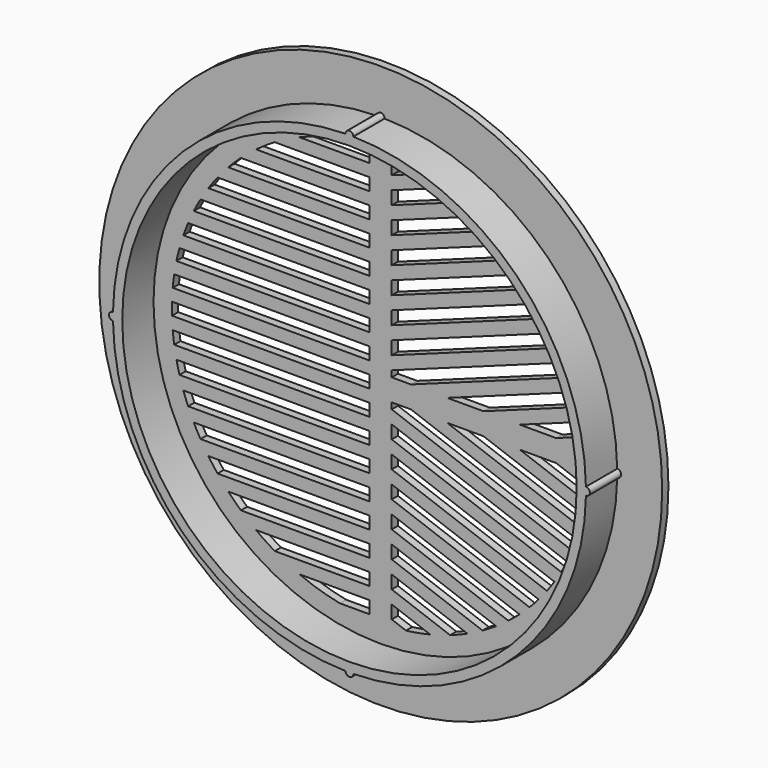
from build123d import *

# Parameters (mm, degrees)
F3_DEPTH      = 25
F2_R          = 58.1248774064
F4_DEPTH      = 2
F2_R_2        = 72
F5_DEPTH      = 10
F5_DEPTH_BACK = 2
F7_DEPTH      = 2


# Not quite as in the source:
# - ends of sketch curves that miss each other by under 0.0002 mm in the source are joined


with BuildPart() as f3:
    # F2 (on offset) → F3 (new body)
    with BuildSketch(Plane.XZ.offset(-10)):
        with BuildLine():
            Line((-2.8117546, -52.3882112), (-10.4651656881, -52.3882112))
            ThreePointArc((-10.4651656881, -52.3882112), (-2.0290554984, -53.3847103523), (6.4583568386, -53.0314434327))
            Line((6.4583568386, -53.0314434327), (2.8133294, -51.7046972))
            Line((2.8133294, -51.7046972), (2.8133294, -48.3271576))
            Line((2.8133294, -48.3271576), (12.6439208004, -51.9054489665))
            ThreePointArc((12.6439208004, -51.9054489665), (15.218427268, -51.2098021584), (17.7550108574, -50.3865453774))
            Line((17.7550108574, -50.3865453774), (2.8133294, -44.9481956))
            Line((2.8133294, -44.9481956), (2.8133294, -41.5692336))
            Line((2.8133294, -41.5692336), (22.1596901051, -48.610621268))
            ThreePointArc((22.1596901051, -48.610621268), (24.1217019206, -47.6674717398), (26.0436606582, -46.6451723669))
            Line((26.0436606582, -46.6451723669), (2.8133294, -38.1905256))
            Line((2.8133294, -38.1905256), (2.8133294, -34.8115636))
            Line((2.8133294, -34.8115636), (29.5155011347, -44.529535798))
            ThreePointArc((29.5155011347, -44.529535798), (31.0993092601, -43.4382012652), (32.6428059495, -42.2905614217))
            Line((32.6428059495, -42.2905614217), (2.8133294, -31.4323476))
            Line((2.8133294, -31.4323476), (2.8133294, -28.0533856))
            Line((2.8133294, -28.0533856), (35.4767217693, -39.9430416734))
            ThreePointArc((35.4767217693, -39.9430416734), (36.7835304475, -38.7429510161), (38.0497674642, -37.500127487))
            Line((38.0497674642, -37.500127487), (2.8133294, -24.6744236))
            Line((2.8133294, -24.6744236), (2.8133294, -21.2969856))
            Line((2.8133294, -21.2969856), (40.3860770749, -34.9715476368))
            ThreePointArc((40.3860770749, -34.9715476368), (41.4655782018, -33.6845690192), (42.5040845927, -32.3642883214))
            Line((42.5040845927, -32.3642883214), (2.8133294, -17.9180236))
            Line((2.8133294, -17.9180236), (2.8133294, -14.5390616))
            Line((2.8133294, -14.5390616), (44.4188112616, -29.6818727798))
            ThreePointArc((44.4188112616, -29.6818727798), (45.3001399367, -28.3185749524), (46.1396401032, -26.9291287784))
            Line((46.1396401032, -26.9291287784), (2.8133294, -11.1603536))
            Line((2.8133294, -11.1603536), (2.8133294, -7.7808836))
            Line((2.8133294, -7.7808836), (47.6735638969, -24.109659288))
            ThreePointArc((47.6735638969, -24.109659288), (48.3716674827, -22.6765550857), (49.0267027126, -21.2232605117))
            Line((49.0267027126, -21.2232605117), (2.8133294, -4.4021756))
            Line((2.8133294, -4.4021756), (2.8133294, -2.8131516))
            Line((2.8133294, -2.8131516), (7.7274674, -2.8131516))
            Line((7.7274674, -2.8131516), (50.2014340828, -18.271846695))
            ThreePointArc((50.2014340828, -18.271846695), (50.722459913, -16.7712976835), (51.1986446, -15.2559220219))
            Line((51.1986446, -15.2559220219), (17.0096434, -2.8131516))
            Line((17.0096434, -2.8131516), (26.2938514, -2.8131516))
            Line((26.2938514, -2.8131516), (52.0175000452, -12.1747301681))
            ThreePointArc((52.0175000452, -12.1747301681), (52.3597146995, -10.6068205513), (52.654680648, -9.0293394816))
            Line((52.654680648, -9.0293394816), (35.5760274, -2.8131516))
            Line((35.5760274, -2.8131516), (44.8599814, -2.8131516))
            Line((44.8599814, -2.8131516), (53.1059491143, -5.8139946928))
            ThreePointArc((53.1059491143, -5.8139946928), (53.3438708851, -2.9113235155), (53.4232567859, 0))
            ThreePointArc((53.4232567859, 0), (53.3438698733, 2.9113420537), (53.1059450733, 5.814031604))
            Line((53.1059450733, 5.814031604), (44.8599814, 2.8119324))
            Line((44.8599814, 2.8119324), (35.5760274, 2.8119324))
            Line((35.5760274, 2.8119324), (52.6549590226, 9.0277159873))
            ThreePointArc((52.6549590226, 9.0277159873), (52.3598738539, 10.6060348678), (52.0174900396, 12.1747729176))
            Line((52.0174900396, 12.1747729176), (26.2938514, 2.8119324))
            Line((26.2938514, 2.8119324), (17.0096434, 2.8119324))
            Line((17.0096434, 2.8119324), (51.1986319495, 15.2559644767))
            ThreePointArc((51.1986319495, 15.2559644767), (50.7224085028, 16.7714531659), (50.2013372139, 18.2721128376))
            Line((50.2013372139, 18.2721128376), (7.7274674, 2.8119324))
            Line((7.7274674, 2.8119324), (2.8133294, 2.8119324))
            Line((2.8133294, 2.8119324), (2.8133294, 4.4022264))
            Line((2.8133294, 4.4022264), (49.0268732907, 21.222866464))
            ThreePointArc((49.0268732907, 21.222866464), (48.3720536469, 22.6757313354), (47.6741912545, 24.1084187338))
            Line((47.6741912545, 24.1084187338), (2.8133294, 7.7811884))
            Line((2.8133294, 7.7811884), (2.8133294, 11.1598964))
            Line((2.8133294, 11.1598964), (46.1394942326, 26.9293787076))
            ThreePointArc((46.1394942326, 26.9293787076), (45.3001153405, 28.318614298), (44.4189204817, 29.6817093318))
            Line((44.4189204817, 29.6817093318), (2.8133294, 14.5388584))
            Line((2.8133294, 14.5388584), (2.8133294, 17.9178204))
            Line((2.8133294, 17.9178204), (42.5040547328, 32.3643275364))
            ThreePointArc((42.5040547328, 32.3643275364), (41.4655480706, 33.6846061106), (40.3860467755, 34.9715826274))
            Line((40.3860467755, 34.9715826274), (2.8133294, 21.2952584))
            Line((2.8133294, 21.2952584), (2.8133294, 24.6744744))
            Line((2.8133294, 24.6744744), (38.0499142876, 37.4999785109))
            ThreePointArc((38.0499142876, 37.4999785109), (36.783684661, 38.7428046013), (35.4768833619, 39.942898149))
            Line((35.4768833619, 39.942898149), (2.8133294, 28.0534364))
            Line((2.8133294, 28.0534364), (2.8133294, 31.4323984))
            Line((2.8133294, 31.4323984), (32.6429839509, 42.2904240271))
            ThreePointArc((32.6429839509, 42.2904240271), (31.0993770857, 43.4381527059), (29.5154527684, 44.5295678566))
            Line((29.5154527684, 44.5295678566), (2.8133294, 34.8113604))
            Line((2.8133294, 34.8113604), (2.8133294, 38.1903224))
            Line((2.8133294, 38.1903224), (26.04388098, 46.6450493527))
            ThreePointArc((26.04388098, 46.6450493527), (24.1219360197, 47.6673532753), (22.1599379618, 48.610508279))
            Line((22.1599379618, 48.610508279), (2.8133294, 41.5690304))
            Line((2.8133294, 41.5690304), (2.8133294, 44.9479924))
            Line((2.8133294, 44.9479924), (17.7553997833, 50.3864083276))
            ThreePointArc((17.7553997833, 50.3864083276), (15.2185413933, 51.2097682427), (12.643751501, 51.9054902067))
            Line((12.643751501, 51.9054902067), (2.8133294, 48.3259384))
            Line((2.8133294, 48.3259384), (2.8133294, 51.7046464))
            Line((2.8133294, 51.7046464), (6.4589618961, 53.0313697432))
            ThreePointArc((6.4589618961, 53.0313697432), (-2.0327661079, 53.3845691897), (-10.4730459901, 52.3866364))
            Line((-10.4730459901, 52.3866364), (-2.8117546, 52.3866364))
            Line((-2.8117546, 52.3866364), (-2.8117546, 49.2116364))
            Line((-2.8117546, 49.2116364), (-20.7908443419, 49.2116364))
            ThreePointArc((-20.7908443419, 49.2116364), (-24.0004032321, 47.728660261), (-27.104842272, 46.0366364))
            Line((-27.104842272, 46.0366364), (-2.8117546, 46.0366364))
            Line((-2.8117546, 46.0366364), (-2.8117546, 42.8616364))
            Line((-2.8117546, 42.8616364), (-31.8892535305, 42.8616364))
            ThreePointArc((-31.8892535305, 42.8616364), (-33.8635191157, 41.3195648418), (-35.7633227884, 39.6866364))
            Line((-35.7633227884, 39.6866364), (-2.8117546, 39.6866364))
            Line((-2.8117546, 39.6866364), (-2.8117546, 36.5116364))
            Line((-2.8117546, 36.5116364), (-38.9992919552, 36.5116364))
            ThreePointArc((-38.9992919552, 36.5116364), (-40.4037524944, 34.9511251605), (-41.7458146303, 33.3366364))
            Line((-41.7458146303, 33.3366364), (-2.8117546, 33.3366364))
            Line((-2.8117546, 33.3366364), (-2.8117546, 30.1616364))
            Line((-2.8117546, 30.1616364), (-44.0944447214, 30.1616364))
            ThreePointArc((-44.0944447214, 30.1616364), (-45.1281672323, 28.5918325377), (-46.1060280379, 26.9866364))
            Line((-46.1060280379, 26.9866364), (-2.8117546, 26.9866364))
            Line((-2.8117546, 26.9866364), (-2.8117546, 23.8116364))
            Line((-2.8117546, 23.8116364), (-47.8231150969, 23.8116364))
            ThreePointArc((-47.8231150969, 23.8116364), (-48.5757557209, 22.2360140709), (-49.2765015368, 20.6366364))
            Line((-49.2765015368, 20.6366364), (-2.8117546, 20.6366364))
            Line((-2.8117546, 20.6366364), (-2.8117546, 17.4616364))
            Line((-2.8117546, 17.4616364), (-50.4889653276, 17.4616364))
            ThreePointArc((-50.4889653276, 17.4616364), (-51.0079586216, 15.8818299598), (-51.4775328273, 14.2866364))
            Line((-51.4775328273, 14.2866364), (-2.8117546, 14.2866364))
            Line((-2.8117546, 14.2866364), (-2.8117546, 11.1116364))
            Line((-2.8117546, 11.1116364), (-52.2549127081, 11.1116364))
            ThreePointArc((-52.2549127081, 11.1116364), (-52.5666470955, 9.5284825), (-52.8304284316, 7.9366364))
            Line((-52.8304284316, 7.9366364), (-2.8117546, 7.9366364))
            Line((-2.8117546, 7.9366364), (-2.8117546, 4.7616364))
            Line((-2.8117546, 4.7616364), (-53.2106303704, 4.7616364))
            ThreePointArc((-53.2106303704, 4.7616364), (-53.3287941262, 3.1755444663), (-53.399690502, 1.5866379243))
            Line((-53.399690502, 1.5866379243), (-2.8117546, 1.5866364))
            Line((-2.8117546, 1.5866364), (-2.8117546, -1.5883636))
            Line((-2.8117546, -1.5883636), (-53.3996392, -1.5883636))
            ThreePointArc((-53.3996392, -1.5883636), (-53.3286912488, -3.1772716764), (-53.2104757809, -4.7633636))
            Line((-53.2104757809, -4.7633636), (-2.8117546, -4.7633636))
            Line((-2.8117546, -4.7633636), (-2.8117546, -7.9383636))
            Line((-2.8117546, -7.9383636), (-52.8301689281, -7.9383636))
            ThreePointArc((-52.8301689281, -7.9383636), (-52.5663338333, -9.53021054), (-52.2545454014, -11.1133636))
            Line((-52.2545454014, -11.1133636), (-2.8117546, -11.1133636))
            Line((-2.8117546, -11.1133636), (-2.8117546, -14.2883636))
            Line((-2.8117546, -14.2883636), (-51.4770534437, -14.2883636))
            ThreePointArc((-51.4770534437, -14.2883636), (-51.0074204976, -15.8835581593), (-50.4883679414, -17.4633636))
            Line((-50.4883679414, -17.4633636), (-2.8117546, -17.4633636))
            Line((-2.8117546, -17.4633636), (-2.8117546, -20.6383636))
            Line((-2.8117546, -20.6383636), (-49.2757781626, -20.6383636))
            ThreePointArc((-49.2757781626, -20.6383636), (-48.5749644416, -22.2377425813), (-47.8222550668, -23.8133636))
            Line((-47.8222550668, -23.8133636), (-2.8117546, -23.8133636))
            Line((-2.8117546, -23.8133636), (-2.8117546, -26.9883636))
            Line((-2.8117546, -26.9883636), (-46.1050170351, -26.9883636))
            ThreePointArc((-46.1050170351, -26.9883636), (-45.127071662, -28.5935616675), (-44.0932632264, -30.1633636))
            Line((-44.0932632264, -30.1633636), (-2.8117546, -30.1633636))
            Line((-2.8117546, -30.1633636), (-2.8117546, -33.3383636))
            Line((-2.8117546, -33.3383636), (-41.7444352949, -33.3383636))
            ThreePointArc((-41.7444352949, -33.3383636), (-40.4022554344, -34.9528556978), (-38.9976748567, -36.5133636))
            Line((-38.9976748567, -36.5133636), (-2.8117546, -36.5133636))
            Line((-2.8117546, -36.5133636), (-2.8117546, -39.6881096))
            Line((-2.8117546, -39.6881096), (-35.7616879075, -39.6881096))
            ThreePointArc((-35.7616879075, -39.6881096), (-33.8617135671, -41.3210445162), (-31.8872733396, -42.8631096))
            Line((-31.8872733396, -42.8631096), (-2.8117546, -42.8631096))
            Line((-2.8117546, -42.8631096), (-2.8117546, -46.0381096))
            Line((-2.8117546, -46.0381096), (-27.1023399373, -46.0381096))
            ThreePointArc((-27.1023399373, -46.0381096), (-23.9972982866, -47.7302214594), (-20.7871164186, -49.2132112))
            Line((-20.7871164186, -49.2132112), (-2.8117546, -49.2132112))
            Line((-2.8117546, -49.2132112), (-2.8117546, -52.3882112))
        make_face()
    extrude(amount=F3_DEPTH)


with BuildPart() as f4:
    # F2 (on offset) → F4 (new body)
    with BuildSketch(Plane.XZ.offset(-10)):
        Circle(F2_R)
        with BuildLine():
            ThreePointArc((6.4583568386, -53.0314434327), (-2.0290554984, -53.3847103523), (-10.4651656881, -52.3882112))
            ThreePointArc((-10.4651656881, -52.3882112), (-15.7065731612, -51.0621966346), (-20.7871164186, -49.2132112))
            ThreePointArc((-20.7871164186, -49.2132112), (-23.9972982866, -47.7302214594), (-27.1023399373, -46.0381096))
            ThreePointArc((-27.1023399373, -46.0381096), (-29.5374977764, -44.514947947), (-31.8872733396, -42.8631096))
            ThreePointArc((-31.8872733396, -42.8631096), (-33.8617135671, -41.3210445162), (-35.7616879075, -39.6881096))
            ThreePointArc((-35.7616879075, -39.6881096), (-37.4133710493, -38.1350761419), (-38.9976748567, -36.5133636))
            ThreePointArc((-38.9976748567, -36.5133636), (-40.4022554344, -34.9528556978), (-41.7444352949, -33.3383636))
            ThreePointArc((-41.7444352949, -33.3383636), (-42.9481987761, -31.7725760288), (-44.0932632264, -30.1633636))
            ThreePointArc((-44.0932632264, -30.1633636), (-45.127071662, -28.5935616675), (-46.1050170351, -26.9883636))
            ThreePointArc((-46.1050170351, -26.9883636), (-46.9904593229, -25.4153712985), (-47.8222550668, -23.8133636))
            ThreePointArc((-47.8222550668, -23.8133636), (-48.5749644416, -22.2377425813), (-49.2757781626, -20.6383636))
            ThreePointArc((-49.2757781626, -20.6383636), (-49.9073278008, -19.0605088442), (-50.4883679414, -17.4633636))
            ThreePointArc((-50.4883679414, -17.4633636), (-51.0074204976, -15.8835581593), (-51.4770534437, -14.2883636))
            ThreePointArc((-51.4770534437, -14.2883636), (-51.8900887067, -12.7068115443), (-52.2545454014, -11.1133636))
            ThreePointArc((-52.2545454014, -11.1133636), (-52.5663338333, -9.53021054), (-52.8301689281, -7.9383636))
            ThreePointArc((-52.8301689281, -7.9383636), (-53.0440829766, -6.3537096874), (-53.2104757809, -4.7633636))
            ThreePointArc((-53.2104757809, -4.7633636), (-53.3286912488, -3.1772716764), (-53.3996392, -1.5883636))
            ThreePointArc((-53.3996392, -1.5883636), (-53.423256779, -0.000863219), (-53.399690502, 1.5866379243))
            ThreePointArc((-53.399690502, 1.5866379243), (-53.3287941262, 3.1755444663), (-53.2106303704, 4.7616364))
            ThreePointArc((-53.2106303704, 4.7616364), (-53.0442899303, 6.3519816911), (-52.8304284316, 7.9366364))
            ThreePointArc((-52.8304284316, 7.9366364), (-52.5666470955, 9.5284825), (-52.2549127081, 11.1116364))
            ThreePointArc((-52.2549127081, 11.1116364), (-51.8905118537, 12.7050834384), (-51.4775328273, 14.2866364))
            ThreePointArc((-51.4775328273, 14.2866364), (-51.0079586216, 15.8818299598), (-50.4889653276, 17.4616364))
            ThreePointArc((-50.4889653276, 17.4616364), (-49.9079878468, 19.0587805144), (-49.2765015368, 20.6366364))
            ThreePointArc((-49.2765015368, 20.6366364), (-48.5757557209, 22.2360140709), (-47.8231150969, 23.8116364))
            ThreePointArc((-47.8231150969, 23.8116364), (-46.9913943053, 25.4136425342), (-46.1060280379, 26.9866364))
            ThreePointArc((-46.1060280379, 26.9866364), (-45.1281672323, 28.5918325377), (-44.0944447214, 30.1616364))
            ThreePointArc((-44.0944447214, 30.1616364), (-42.9494783163, 31.7708463528), (-41.7458146303, 33.3366364))
            ThreePointArc((-41.7458146303, 33.3366364), (-40.4037524944, 34.9511251605), (-38.9992919552, 36.5116364))
            ThreePointArc((-38.9992919552, 36.5116364), (-37.4150009632, 38.1334770056), (-35.7633227884, 39.6866364))
            ThreePointArc((-35.7633227884, 39.6866364), (-33.8635191157, 41.3195648418), (-31.8892535305, 42.8616364))
            ThreePointArc((-31.8892535305, 42.8616364), (-29.5397358001, 44.5134628453), (-27.104842272, 46.0366364))
            ThreePointArc((-27.104842272, 46.0366364), (-24.0004032321, 47.728660261), (-20.7908443419, 49.2116364))
            ThreePointArc((-20.7908443419, 49.2116364), (-15.7123475624, 51.0604200893), (-10.4730459901, 52.3866364))
            ThreePointArc((-10.4730459901, 52.3866364), (-2.0327661079, 53.3845691897), (6.4589618961, 53.0313697432))
            ThreePointArc((6.4589618961, 53.0313697432), (9.5679316451, 52.5594810634), (12.643751501, 51.9054902067))
            ThreePointArc((12.643751501, 51.9054902067), (15.2185413933, 51.2097682427), (17.7553997833, 50.3864083276))
            ThreePointArc((17.7553997833, 50.3864083276), (19.9774122967, 49.5474253977), (22.1599379618, 48.610508279))
            ThreePointArc((22.1599379618, 48.610508279), (24.1219360197, 47.6673532753), (26.04388098, 46.6450493527))
            ThreePointArc((26.04388098, 46.6450493527), (27.7997968901, 45.620342595), (29.5154527684, 44.5295678566))
            ThreePointArc((29.5154527684, 44.5295678566), (31.0993770857, 43.4381527059), (32.6429839509, 42.2904240271))
            ThreePointArc((32.6429839509, 42.2904240271), (34.0801525835, 41.1410690855), (35.4768833619, 39.942898149))
            ThreePointArc((35.4768833619, 39.942898149), (36.783684661, 38.7428046013), (38.0499142876, 37.4999785109))
            ThreePointArc((38.0499142876, 37.4999785109), (39.2383510536, 36.2546020832), (40.3860467755, 34.9715826274))
            ThreePointArc((40.3860467755, 34.9715826274), (41.4655480706, 33.6846061106), (42.5040547328, 32.3643275364))
            ThreePointArc((42.5040547328, 32.3643275364), (43.4821804323, 31.0377890719), (44.4189204817, 29.6817093318))
            ThreePointArc((44.4189204817, 29.6817093318), (45.3001153405, 28.318614298), (46.1394942326, 26.9293787075))
            ThreePointArc((46.1394942326, 26.9293787075), (46.9280443867, 25.530433127), (47.6741912545, 24.1084187338))
            ThreePointArc((47.6741912545, 24.1084187338), (48.3720536469, 22.6757313354), (49.0268732907, 21.222866464))
            ThreePointArc((49.0268732907, 21.222866464), (49.6360370772, 19.7562189927), (50.2013372139, 18.2721128376))
            ThreePointArc((50.2013372139, 18.2721128376), (50.7224085028, 16.7714531659), (51.1986319495, 15.2559644767))
            ThreePointArc((51.1986319495, 15.2559644767), (51.6310506863, 13.7214784423), (52.0174900396, 12.1747729176))
            ThreePointArc((52.0174900396, 12.1747729176), (52.3598738539, 10.6060348678), (52.6549590226, 9.0277159873))
            ThreePointArc((52.6549590226, 9.0277159873), (52.9048594235, 7.4242989565), (53.1059450733, 5.814031604))
            ThreePointArc((53.1059450733, 5.814031604), (53.3438698733, 2.9113420537), (53.4232567859, 0))
            ThreePointArc((53.4232567859, 0), (53.3438708851, -2.9113235155), (53.1059491143, -5.8139946928))
            ThreePointArc((53.1059491143, -5.8139946928), (52.9047475417, -7.4250961718), (52.654680648, -9.0293394816))
            ThreePointArc((52.654680648, -9.0293394816), (52.3597146995, -10.6068205513), (52.0175000452, -12.1747301681))
            ThreePointArc((52.0175000452, -12.1747301681), (51.6310620137, -13.7214358196), (51.1986446, -15.2559220219))
            ThreePointArc((51.1986446, -15.2559220219), (50.722459913, -16.7712976835), (50.2014340828, -18.271846695))
            ThreePointArc((50.2014340828, -18.271846695), (49.6360100517, -19.7562868921), (49.0267027126, -21.2232605117))
            ThreePointArc((49.0267027126, -21.2232605117), (48.3716674827, -22.6765550857), (47.6735638969, -24.109659288))
            ThreePointArc((47.6735638969, -24.109659288), (46.9277813586, -25.5309165988), (46.1396401032, -26.9291287784))
            ThreePointArc((46.1396401032, -26.9291287784), (45.3001399367, -28.3185749524), (44.4188112616, -29.6818727798))
            ThreePointArc((44.4188112616, -29.6818727798), (43.4821376454, -31.0378490138), (42.5040845927, -32.3642883214))
            ThreePointArc((42.5040845927, -32.3642883214), (41.4655782018, -33.6845690192), (40.3860770749, -34.9715476368))
            ThreePointArc((40.3860770749, -34.9715476368), (39.2382957856, -36.2546618997), (38.0497674642, -37.500127487))
            ThreePointArc((38.0497674642, -37.500127487), (36.7835304475, -38.7429510161), (35.4767217693, -39.9430416734))
            ThreePointArc((35.4767217693, -39.9430416734), (34.0799827817, -41.1412097442), (32.6428059495, -42.2905614217))
            ThreePointArc((32.6428059495, -42.2905614217), (31.0993092601, -43.4382012652), (29.5155011347, -44.529535798))
            ThreePointArc((29.5155011347, -44.529535798), (27.7997139249, -45.6203931517), (26.0436606582, -46.6451723669))
            ThreePointArc((26.0436606582, -46.6451723669), (24.1217019206, -47.6674717398), (22.1596901051, -48.610621268))
            ThreePointArc((22.1596901051, -48.610621268), (19.9770947548, -49.5475534287), (17.7550108574, -50.3865453774))
            ThreePointArc((17.7550108574, -50.3865453774), (15.218427268, -51.2098021584), (12.6439208004, -51.9054489665))
            ThreePointArc((12.6439208004, -51.9054489665), (9.5677175248, -52.5595200414), (6.4583568386, -53.0314434327))
        make_face(mode=Mode.SUBTRACT)
        with BuildLine():
            Line((-2.8117546, -52.3882112), (-10.4651656881, -52.3882112))
            ThreePointArc((-10.4651656881, -52.3882112), (-2.0290554984, -53.3847103523), (6.4583568386, -53.0314434327))
            Line((6.4583568386, -53.0314434327), (2.8133294, -51.7046972))
            Line((2.8133294, -51.7046972), (2.8133294, -48.3271576))
            Line((2.8133294, -48.3271576), (12.6439208004, -51.9054489665))
            ThreePointArc((12.6439208004, -51.9054489665), (15.218427268, -51.2098021584), (17.7550108574, -50.3865453774))
            Line((17.7550108574, -50.3865453774), (2.8133294, -44.9481956))
            Line((2.8133294, -44.9481956), (2.8133294, -41.5692336))
            Line((2.8133294, -41.5692336), (22.1596901051, -48.610621268))
            ThreePointArc((22.1596901051, -48.610621268), (24.1217019206, -47.6674717398), (26.0436606582, -46.6451723669))
            Line((26.0436606582, -46.6451723669), (2.8133294, -38.1905256))
            Line((2.8133294, -38.1905256), (2.8133294, -34.8115636))
            Line((2.8133294, -34.8115636), (29.5155011347, -44.529535798))
            ThreePointArc((29.5155011347, -44.529535798), (31.0993092601, -43.4382012652), (32.6428059495, -42.2905614217))
            Line((32.6428059495, -42.2905614217), (2.8133294, -31.4323476))
            Line((2.8133294, -31.4323476), (2.8133294, -28.0533856))
            Line((2.8133294, -28.0533856), (35.4767217693, -39.9430416734))
            ThreePointArc((35.4767217693, -39.9430416734), (36.7835304475, -38.7429510161), (38.0497674642, -37.500127487))
            Line((38.0497674642, -37.500127487), (2.8133294, -24.6744236))
            Line((2.8133294, -24.6744236), (2.8133294, -21.2969856))
            Line((2.8133294, -21.2969856), (40.3860770749, -34.9715476368))
            ThreePointArc((40.3860770749, -34.9715476368), (41.4655782018, -33.6845690192), (42.5040845927, -32.3642883214))
            Line((42.5040845927, -32.3642883214), (2.8133294, -17.9180236))
            Line((2.8133294, -17.9180236), (2.8133294, -14.5390616))
            Line((2.8133294, -14.5390616), (44.4188112616, -29.6818727798))
            ThreePointArc((44.4188112616, -29.6818727798), (45.3001399367, -28.3185749524), (46.1396401032, -26.9291287784))
            Line((46.1396401032, -26.9291287784), (2.8133294, -11.1603536))
            Line((2.8133294, -11.1603536), (2.8133294, -7.7808836))
            Line((2.8133294, -7.7808836), (47.6735638969, -24.109659288))
            ThreePointArc((47.6735638969, -24.109659288), (48.3716674827, -22.6765550857), (49.0267027126, -21.2232605117))
            Line((49.0267027126, -21.2232605117), (2.8133294, -4.4021756))
            Line((2.8133294, -4.4021756), (2.8133294, -2.8131516))
            Line((2.8133294, -2.8131516), (7.7274674, -2.8131516))
            Line((7.7274674, -2.8131516), (50.2014340828, -18.271846695))
            ThreePointArc((50.2014340828, -18.271846695), (50.722459913, -16.7712976835), (51.1986446, -15.2559220219))
            Line((51.1986446, -15.2559220219), (17.0096434, -2.8131516))
            Line((17.0096434, -2.8131516), (26.2938514, -2.8131516))
            Line((26.2938514, -2.8131516), (52.0175000452, -12.1747301681))
            ThreePointArc((52.0175000452, -12.1747301681), (52.3597146995, -10.6068205513), (52.654680648, -9.0293394816))
            Line((52.654680648, -9.0293394816), (35.5760274, -2.8131516))
            Line((35.5760274, -2.8131516), (44.8599814, -2.8131516))
            Line((44.8599814, -2.8131516), (53.1059491143, -5.8139946928))
            ThreePointArc((53.1059491143, -5.8139946928), (53.3438708851, -2.9113235155), (53.4232567859, 0))
            ThreePointArc((53.4232567859, 0), (53.3438698733, 2.9113420537), (53.1059450733, 5.814031604))
            Line((53.1059450733, 5.814031604), (44.8599814, 2.8119324))
            Line((44.8599814, 2.8119324), (35.5760274, 2.8119324))
            Line((35.5760274, 2.8119324), (52.6549590226, 9.0277159873))
            ThreePointArc((52.6549590226, 9.0277159873), (52.3598738539, 10.6060348678), (52.0174900396, 12.1747729176))
            Line((52.0174900396, 12.1747729176), (26.2938514, 2.8119324))
            Line((26.2938514, 2.8119324), (17.0096434, 2.8119324))
            Line((17.0096434, 2.8119324), (51.1986319495, 15.2559644767))
            ThreePointArc((51.1986319495, 15.2559644767), (50.7224085028, 16.7714531659), (50.2013372139, 18.2721128376))
            Line((50.2013372139, 18.2721128376), (7.7274674, 2.8119324))
            Line((7.7274674, 2.8119324), (2.8133294, 2.8119324))
            Line((2.8133294, 2.8119324), (2.8133294, 4.4022264))
            Line((2.8133294, 4.4022264), (49.0268732907, 21.222866464))
            ThreePointArc((49.0268732907, 21.222866464), (48.3720536469, 22.6757313354), (47.6741912545, 24.1084187338))
            Line((47.6741912545, 24.1084187338), (2.8133294, 7.7811884))
            Line((2.8133294, 7.7811884), (2.8133294, 11.1598964))
            Line((2.8133294, 11.1598964), (46.1394942326, 26.9293787076))
            ThreePointArc((46.1394942326, 26.9293787076), (45.3001153405, 28.318614298), (44.4189204817, 29.6817093318))
            Line((44.4189204817, 29.6817093318), (2.8133294, 14.5388584))
            Line((2.8133294, 14.5388584), (2.8133294, 17.9178204))
            Line((2.8133294, 17.9178204), (42.5040547328, 32.3643275364))
            ThreePointArc((42.5040547328, 32.3643275364), (41.4655480706, 33.6846061106), (40.3860467755, 34.9715826274))
            Line((40.3860467755, 34.9715826274), (2.8133294, 21.2952584))
            Line((2.8133294, 21.2952584), (2.8133294, 24.6744744))
            Line((2.8133294, 24.6744744), (38.0499142876, 37.4999785109))
            ThreePointArc((38.0499142876, 37.4999785109), (36.783684661, 38.7428046013), (35.4768833619, 39.942898149))
            Line((35.4768833619, 39.942898149), (2.8133294, 28.0534364))
            Line((2.8133294, 28.0534364), (2.8133294, 31.4323984))
            Line((2.8133294, 31.4323984), (32.6429839509, 42.2904240271))
            ThreePointArc((32.6429839509, 42.2904240271), (31.0993770857, 43.4381527059), (29.5154527684, 44.5295678566))
            Line((29.5154527684, 44.5295678566), (2.8133294, 34.8113604))
            Line((2.8133294, 34.8113604), (2.8133294, 38.1903224))
            Line((2.8133294, 38.1903224), (26.04388098, 46.6450493527))
            ThreePointArc((26.04388098, 46.6450493527), (24.1219360197, 47.6673532753), (22.1599379618, 48.610508279))
            Line((22.1599379618, 48.610508279), (2.8133294, 41.5690304))
            Line((2.8133294, 41.5690304), (2.8133294, 44.9479924))
            Line((2.8133294, 44.9479924), (17.7553997833, 50.3864083276))
            ThreePointArc((17.7553997833, 50.3864083276), (15.2185413933, 51.2097682427), (12.643751501, 51.9054902067))
            Line((12.643751501, 51.9054902067), (2.8133294, 48.3259384))
            Line((2.8133294, 48.3259384), (2.8133294, 51.7046464))
            Line((2.8133294, 51.7046464), (6.4589618961, 53.0313697432))
            ThreePointArc((6.4589618961, 53.0313697432), (-2.0327661079, 53.3845691897), (-10.4730459901, 52.3866364))
            Line((-10.4730459901, 52.3866364), (-2.8117546, 52.3866364))
            Line((-2.8117546, 52.3866364), (-2.8117546, 49.2116364))
            Line((-2.8117546, 49.2116364), (-20.7908443419, 49.2116364))
            ThreePointArc((-20.7908443419, 49.2116364), (-24.0004032321, 47.728660261), (-27.104842272, 46.0366364))
            Line((-27.104842272, 46.0366364), (-2.8117546, 46.0366364))
            Line((-2.8117546, 46.0366364), (-2.8117546, 42.8616364))
            Line((-2.8117546, 42.8616364), (-31.8892535305, 42.8616364))
            ThreePointArc((-31.8892535305, 42.8616364), (-33.8635191157, 41.3195648418), (-35.7633227884, 39.6866364))
            Line((-35.7633227884, 39.6866364), (-2.8117546, 39.6866364))
            Line((-2.8117546, 39.6866364), (-2.8117546, 36.5116364))
            Line((-2.8117546, 36.5116364), (-38.9992919552, 36.5116364))
            ThreePointArc((-38.9992919552, 36.5116364), (-40.4037524944, 34.9511251605), (-41.7458146303, 33.3366364))
            Line((-41.7458146303, 33.3366364), (-2.8117546, 33.3366364))
            Line((-2.8117546, 33.3366364), (-2.8117546, 30.1616364))
            Line((-2.8117546, 30.1616364), (-44.0944447214, 30.1616364))
            ThreePointArc((-44.0944447214, 30.1616364), (-45.1281672323, 28.5918325377), (-46.1060280379, 26.9866364))
            Line((-46.1060280379, 26.9866364), (-2.8117546, 26.9866364))
            Line((-2.8117546, 26.9866364), (-2.8117546, 23.8116364))
            Line((-2.8117546, 23.8116364), (-47.8231150969, 23.8116364))
            ThreePointArc((-47.8231150969, 23.8116364), (-48.5757557209, 22.2360140709), (-49.2765015368, 20.6366364))
            Line((-49.2765015368, 20.6366364), (-2.8117546, 20.6366364))
            Line((-2.8117546, 20.6366364), (-2.8117546, 17.4616364))
            Line((-2.8117546, 17.4616364), (-50.4889653276, 17.4616364))
            ThreePointArc((-50.4889653276, 17.4616364), (-51.0079586216, 15.8818299598), (-51.4775328273, 14.2866364))
            Line((-51.4775328273, 14.2866364), (-2.8117546, 14.2866364))
            Line((-2.8117546, 14.2866364), (-2.8117546, 11.1116364))
            Line((-2.8117546, 11.1116364), (-52.2549127081, 11.1116364))
            ThreePointArc((-52.2549127081, 11.1116364), (-52.5666470955, 9.5284825), (-52.8304284316, 7.9366364))
            Line((-52.8304284316, 7.9366364), (-2.8117546, 7.9366364))
            Line((-2.8117546, 7.9366364), (-2.8117546, 4.7616364))
            Line((-2.8117546, 4.7616364), (-53.2106303704, 4.7616364))
            ThreePointArc((-53.2106303704, 4.7616364), (-53.3287941262, 3.1755444663), (-53.399690502, 1.5866379243))
            Line((-53.399690502, 1.5866379243), (-2.8117546, 1.5866364))
            Line((-2.8117546, 1.5866364), (-2.8117546, -1.5883636))
            Line((-2.8117546, -1.5883636), (-53.3996392, -1.5883636))
            ThreePointArc((-53.3996392, -1.5883636), (-53.3286912488, -3.1772716764), (-53.2104757809, -4.7633636))
            Line((-53.2104757809, -4.7633636), (-2.8117546, -4.7633636))
            Line((-2.8117546, -4.7633636), (-2.8117546, -7.9383636))
            Line((-2.8117546, -7.9383636), (-52.8301689281, -7.9383636))
            ThreePointArc((-52.8301689281, -7.9383636), (-52.5663338333, -9.53021054), (-52.2545454014, -11.1133636))
            Line((-52.2545454014, -11.1133636), (-2.8117546, -11.1133636))
            Line((-2.8117546, -11.1133636), (-2.8117546, -14.2883636))
            Line((-2.8117546, -14.2883636), (-51.4770534437, -14.2883636))
            ThreePointArc((-51.4770534437, -14.2883636), (-51.0074204976, -15.8835581593), (-50.4883679414, -17.4633636))
            Line((-50.4883679414, -17.4633636), (-2.8117546, -17.4633636))
            Line((-2.8117546, -17.4633636), (-2.8117546, -20.6383636))
            Line((-2.8117546, -20.6383636), (-49.2757781626, -20.6383636))
            ThreePointArc((-49.2757781626, -20.6383636), (-48.5749644416, -22.2377425813), (-47.8222550668, -23.8133636))
            Line((-47.8222550668, -23.8133636), (-2.8117546, -23.8133636))
            Line((-2.8117546, -23.8133636), (-2.8117546, -26.9883636))
            Line((-2.8117546, -26.9883636), (-46.1050170351, -26.9883636))
            ThreePointArc((-46.1050170351, -26.9883636), (-45.127071662, -28.5935616675), (-44.0932632264, -30.1633636))
            Line((-44.0932632264, -30.1633636), (-2.8117546, -30.1633636))
            Line((-2.8117546, -30.1633636), (-2.8117546, -33.3383636))
            Line((-2.8117546, -33.3383636), (-41.7444352949, -33.3383636))
            ThreePointArc((-41.7444352949, -33.3383636), (-40.4022554344, -34.9528556978), (-38.9976748567, -36.5133636))
            Line((-38.9976748567, -36.5133636), (-2.8117546, -36.5133636))
            Line((-2.8117546, -36.5133636), (-2.8117546, -39.6881096))
            Line((-2.8117546, -39.6881096), (-35.7616879075, -39.6881096))
            ThreePointArc((-35.7616879075, -39.6881096), (-33.8617135671, -41.3210445162), (-31.8872733396, -42.8631096))
            Line((-31.8872733396, -42.8631096), (-2.8117546, -42.8631096))
            Line((-2.8117546, -42.8631096), (-2.8117546, -46.0381096))
            Line((-2.8117546, -46.0381096), (-27.1023399373, -46.0381096))
            ThreePointArc((-27.1023399373, -46.0381096), (-23.9972982866, -47.7302214594), (-20.7871164186, -49.2132112))
            Line((-20.7871164186, -49.2132112), (-2.8117546, -49.2132112))
            Line((-2.8117546, -49.2132112), (-2.8117546, -52.3882112))
        make_face()
    extrude(amount=-F4_DEPTH)



with BuildPart() as f4b:
    # F2 (on offset) → F4, piece 2 (new body)
    with BuildSketch(Plane.XZ.offset(-10)):
        Circle(F2_R_2)
        with BuildLine():
            ThreePointArc((0.9999658487, 60.4917355372), (42.7799602618, 42.7799602618), (60.4917355372, 0.9999658487))
            ThreePointArc((60.4917355372, 0.9999658487), (61.5, 0), (60.4917355372, -0.9999658487))
            ThreePointArc((60.4917355372, -0.9999658487), (42.7799602618, -42.7799602618), (0.9999658487, -60.4917355372))
            ThreePointArc((0.9999658487, -60.4917355372), (0, -61.5), (-0.9999658487, -60.4917355372))
            ThreePointArc((-0.9999658487, -60.4917355372), (-42.7799602618, -42.7799602618), (-60.4917355372, -0.9999658487))
            ThreePointArc((-60.4917355372, -0.9999658487), (-61.5, 0), (-60.4917355372, 0.9999658487))
            ThreePointArc((-60.4917355372, 0.9999658487), (-42.7799602618, 42.7799602618), (-0.9999658487, 60.4917355372))
            ThreePointArc((-0.9999658487, 60.4917355372), (0, 61.5), (0.9999658487, 60.4917355372))
        make_face(mode=Mode.SUBTRACT)
    extrude(amount=-F4_DEPTH)


with BuildPart() as f4_1:
    add(f4.part)

    add(f4b.part)  # F5 merges F4b
    # F2 (on offset) → F5 (join, two sides)
    with BuildSketch(Plane.XZ.offset(-10)) as f5_sk:
        with BuildLine():
            ThreePointArc((60.4917355372, -0.9999658487), (60.497933849, -0.5), (60.5, 0))
            ThreePointArc((60.5, 0), (60.497933849, 0.5), (60.4917355372, 0.9999658487))
            ThreePointArc((60.4917355372, 0.9999658487), (42.7799602618, 42.7799602618), (0.9999658487, 60.4917355372))
            ThreePointArc((0.9999658487, 60.4917355372), (0, 60.5), (-0.9999658487, 60.4917355372))
            ThreePointArc((-0.9999658487, 60.4917355372), (-42.7799602618, 42.7799602618), (-60.4917355372, 0.9999658487))
            ThreePointArc((-60.4917355372, 0.9999658487), (-60.5, 0), (-60.4917355372, -0.9999658487))
            ThreePointArc((-60.4917355372, -0.9999658487), (-42.7799602618, -42.7799602618), (-0.9999658487, -60.4917355372))
            ThreePointArc((-0.9999658487, -60.4917355372), (0, -60.5), (0.9999658487, -60.4917355372))
            ThreePointArc((0.9999658487, -60.4917355372), (42.7799602618, -42.7799602618), (60.4917355372, -0.9999658487))
        make_face()
        Circle(F2_R, mode=Mode.SUBTRACT)
        with BuildLine():
            ThreePointArc((-0.9999658487, 60.4917355372), (0, 60.5), (0.9999658487, 60.4917355372))
            ThreePointArc((0.9999658487, 60.4917355372), (0, 61.5), (-0.9999658487, 60.4917355372))
        make_face()
        with BuildLine():
            ThreePointArc((60.4917355372, 0.9999658487), (60.497933849, 0.5), (60.5, 0))
            ThreePointArc((60.5, 0), (60.497933849, -0.5), (60.4917355372, -0.9999658487))
            ThreePointArc((60.4917355372, -0.9999658487), (61.5, 0), (60.4917355372, 0.9999658487))
        make_face()
        with BuildLine():
            ThreePointArc((-0.9999658487, -60.4917355372), (0, -61.5), (0.9999658487, -60.4917355372))
            ThreePointArc((0.9999658487, -60.4917355372), (0, -60.5), (-0.9999658487, -60.4917355372))
        make_face()
        with BuildLine():
            ThreePointArc((-60.4917355372, -0.9999658487), (-60.5, 0), (-60.4917355372, 0.9999658487))
            ThreePointArc((-60.4917355372, 0.9999658487), (-61.5, 0), (-60.4917355372, -0.9999658487))
        make_face()
    extrude(amount=F5_DEPTH)
    extrude(f5_sk.sketch, amount=-F5_DEPTH_BACK)

    # F2 (on offset) → F7 (join, through all)
    with BuildSketch(Plane.XZ.offset(-10)):
        Circle(F2_R_2)
        with BuildLine():
            ThreePointArc((0.9999658487, 60.4917355372), (42.7799602618, 42.7799602618), (60.4917355372, 0.9999658487))
            ThreePointArc((60.4917355372, 0.9999658487), (61.5, 0), (60.4917355372, -0.9999658487))
            ThreePointArc((60.4917355372, -0.9999658487), (42.7799602618, -42.7799602618), (0.9999658487, -60.4917355372))
            ThreePointArc((0.9999658487, -60.4917355372), (0, -61.5), (-0.9999658487, -60.4917355372))
            ThreePointArc((-0.9999658487, -60.4917355372), (-42.7799602618, -42.7799602618), (-60.4917355372, -0.9999658487))
            ThreePointArc((-60.4917355372, -0.9999658487), (-61.5, 0), (-60.4917355372, 0.9999658487))
            ThreePointArc((-60.4917355372, 0.9999658487), (-42.7799602618, 42.7799602618), (-0.9999658487, 60.4917355372))
            ThreePointArc((-0.9999658487, 60.4917355372), (0, 61.5), (0.9999658487, 60.4917355372))
        make_face(mode=Mode.SUBTRACT)
    extrude(amount=-F7_DEPTH)


solid = f4_1.part
